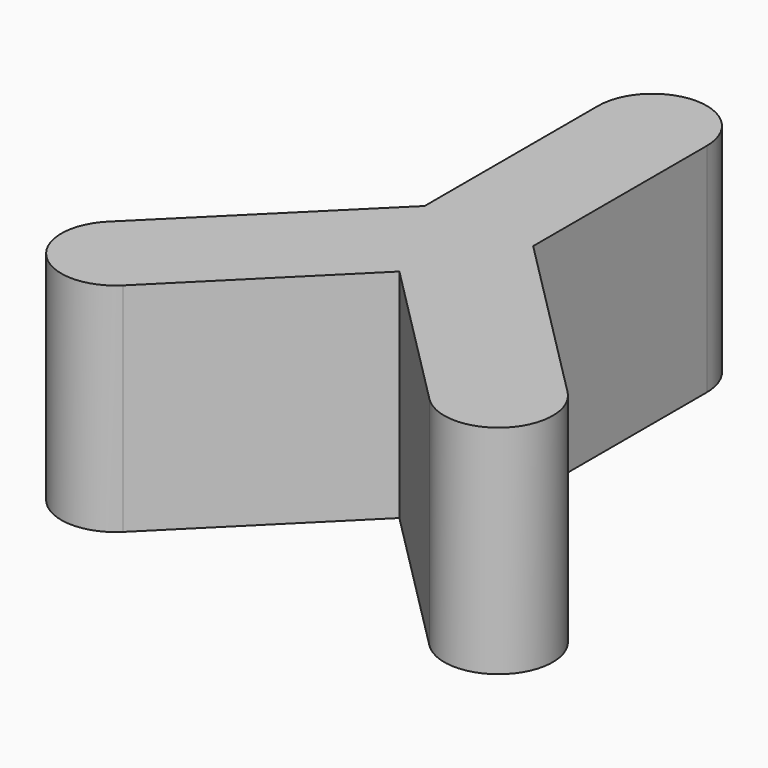
from build123d import *

# Parameters (mm, degrees)
F1_DEPTH = 25.4
F3_DEPTH = 25.4
F5_DEPTH = 114


# Not quite as in the source:
# - an extrude ends at something that could not be found from the text; its depth is read off the source's solid


with BuildPart() as f1:
    # F0 (on Top) → F1 (new body)
    with BuildSketch(Plane.XY):
        Polygon((-25.4796925148, 25.4), (-25.4796925148, 0), (-46.1431506129, -20.4890353627), (-37.1832725133, -29.489623368), (-19.1820965027, -11.569867169), (-1.2623403036, -29.5710431796), (7.7382477017, -20.61116508), (-12.7796925148, 0), (-12.7796925148, 25.4), align=None)
    extrude(amount=F1_DEPTH)

    # F2 (on face) → F3 (join)
    with BuildSketch(Plane.XY.offset(25.4)):
        with BuildLine():
            Line((-25.4796925148, 25.4), (-12.7796925148, 25.4))
            ThreePointArc((-12.7796925148, 25.4), (-19.1296925148, 31.75), (-25.4796925148, 25.4))
        make_face()
        with BuildLine():
            Line((7.7382477017, -20.61116508), (-1.2623403036, -29.5710431796))
            ThreePointArc((-1.2623403036, -29.5710431796), (7.7178927488, -29.5913981325), (7.7382477017, -20.61116508))
        make_face()
        with BuildLine():
            ThreePointArc((-46.1431506129, -20.4890353627), (-46.1635055657, -29.4692684152), (-37.1832725133, -29.489623368))
            Line((-37.1832725133, -29.489623368), (-46.1431506129, -20.4890353627))
        make_face()
    extrude(amount=-F3_DEPTH)

    # F4 (on face) → F5 (cut, through all)
    with BuildSketch(Plane.XY.offset(25.4)):
        with BuildLine():
            Line((-42.5259842963, -16.9024019821), (-40.6344192228, -15.0268038369))
            ThreePointArc((-40.6344192228, -15.0268038369), (-41.6786510297, -15.8653155428), (-42.5259842963, -16.9024019821))
        make_face()
        with BuildLine():
            ThreePointArc((-32.6380296989, -24.9649388112), (-31.2402342157, -22.88066907), (-30.7492439593, -20.4195837129))
            ThreePointArc((-30.7492439593, -20.4195837129), (-34.0912883888, -14.7893358325), (-40.6344192228, -15.0268038369))
            Line((-40.6344192228, -15.0268038369), (-42.5259842963, -16.9024019821))
            ThreePointArc((-42.5259842963, -16.9024019821), (-41.2158295319, -25.3902171382), (-32.6380296989, -24.9649388112))
        make_face()
        with BuildLine():
            ThreePointArc((3.3359301315, -18.6069775374), (2.8926555851, -16.371867323), (1.6299325028, -14.4750962741))
            ThreePointArc((1.6299325028, -14.4750962741), (-7.9341003982, -20.8420877519), (3.3359301315, -18.6069775374))
        make_face()
    extrude(amount=F5_DEPTH, mode=Mode.SUBTRACT)


solid = f1.part
